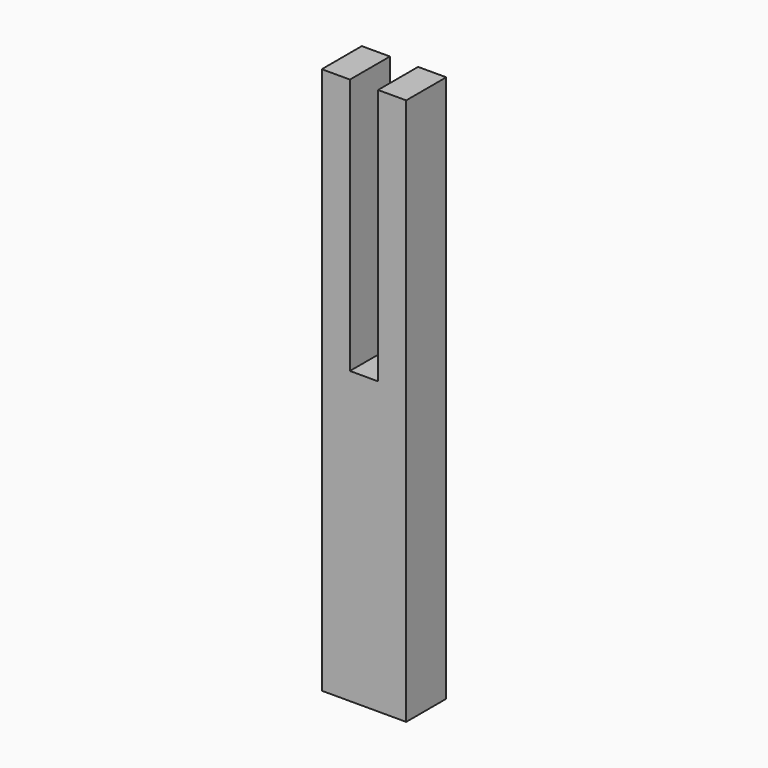
from build123d import *

# Parameters (mm, degrees)
F1_DEPTH      = 16
F1_DEPTH_BACK = 16


# Not quite as in the source:
# - a feature names something its author has since deleted; it is built from what else it names


with BuildPart() as f1:
    # F0 (on Front) → F1 (new body, two sides)
    with BuildSketch(Plane.XZ) as f1_sk:
        Polygon((-9, 77.4134680122), (-27, 77.4134680122), (-27, -272.5865319878), (-9, -272.5865319878), (9, -272.5865319878), (27, -272.5865319878), (27, 77.4134680122), (9, 77.4134680122), (9, -86.6605598913), (-9, -86.6605598913), align=None)
    extrude(amount=F1_DEPTH)
    extrude(f1_sk.sketch, amount=-F1_DEPTH_BACK)


solid = f1.part
